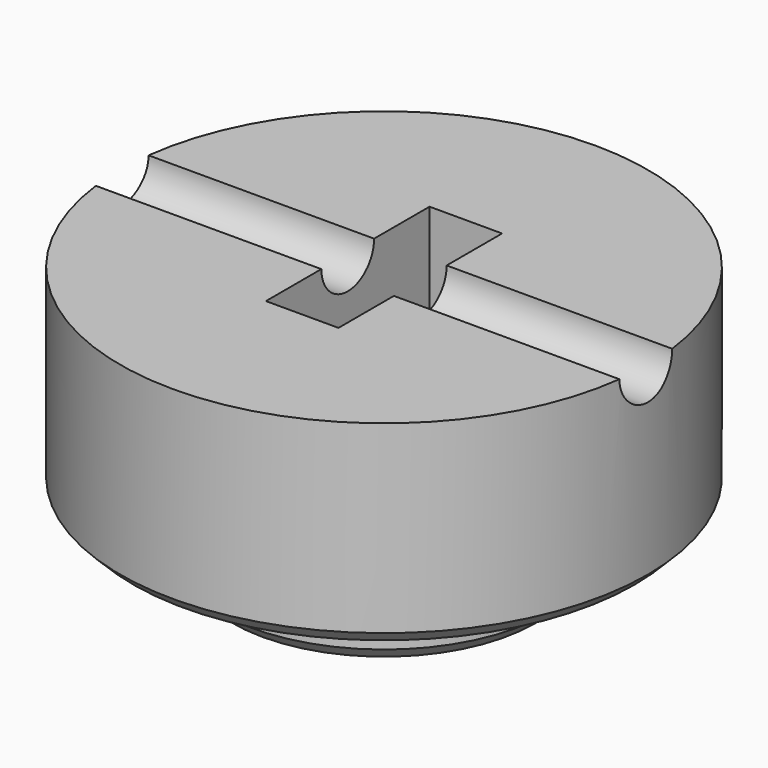
from build123d import *

# Parameters (mm, degrees)
F0_R     = 4
F1_DEPTH = 3
F2_R     = 2.5
F3_DEPTH = 1
F4_R     = 0.5
F5_DEPTH = 9
F6_W     = 1.1
F6_H     = 1.05
F6_H_2   = 1
F7_DEPTH = 4.001
F8_SIZE  = 0.2


# Not quite as in the source:
# - a feature names something its author has since deleted; it is built from what else it names


with BuildPart() as f1:
    # F0 (on Top) → F1 (new body)
    with BuildSketch(Plane.XY):
        Circle(F0_R)
    extrude(amount=-F1_DEPTH)

    # F2 (on face) → F3 (join)
    with BuildSketch(Plane(origin=(0, 0, -3), x_dir=(1, 0, 0), z_dir=(0, 0, -1))):
        Circle(F2_R)
    extrude(amount=F3_DEPTH)

    # F4 (on Right) → F5 (cut, symmetric)
    with BuildSketch(Plane.YZ):
        Circle(F4_R)
    extrude(amount=F5_DEPTH, both=True, mode=Mode.SUBTRACT)

    # F6 (on face) → F7 (cut, through all)
    with BuildSketch(Plane.XY):
        with Locations((0, -1.025)):
            Rectangle(F6_W, F6_H)
        Rectangle(F6_W, F6_H_2)
        with Locations((0, 1.025)):
            Rectangle(F6_W, F6_H)
    extrude(amount=-F7_DEPTH, mode=Mode.SUBTRACT)

    # F8
    f8_edges = [f1.edges().sort_by_distance(p)[0] for p in [
        (-4, 0, -3),
        (-2.5, 0, -4),
    ]]
    chamfer(f8_edges, length=F8_SIZE)


solid = f1.part
